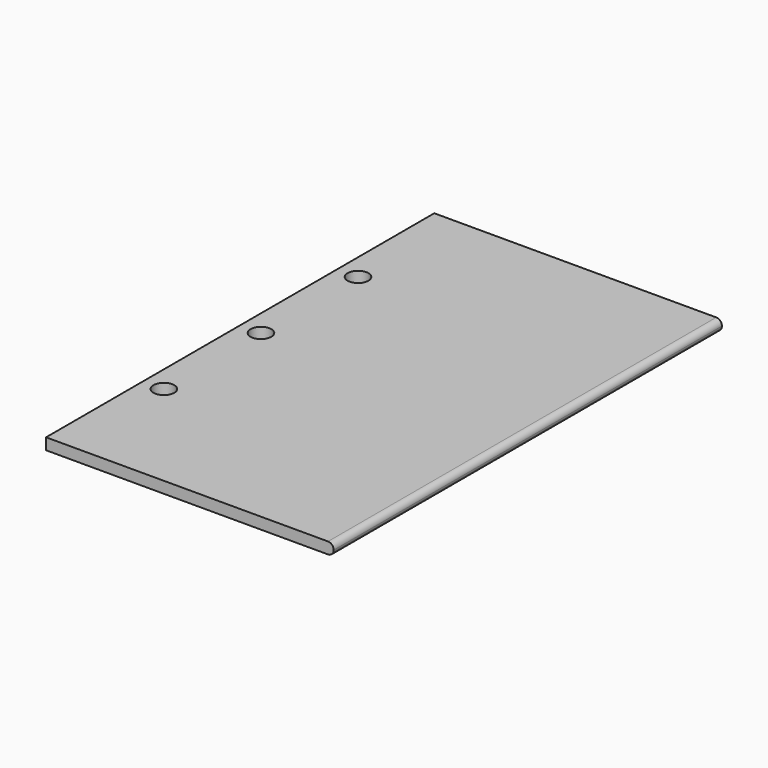
from build123d import *

# Parameters (mm, degrees)
F0_W     = 830
F0_H     = 1400
F1_DEPTH = 33
F2_R     = 16.49999
F4_D     = 60


# Not quite as in the source:
# - a fillet or chamfer is up to 0.001 mm smaller than in the source, because OpenCascade refuses the exact size


with BuildPart() as f1:
    # F0 (on Top) → F1 (new body)
    with BuildSketch(Plane.XY):
        with Locations((354.4717663527, -700)):
            Rectangle(F0_W, F0_H)
    extrude(amount=F1_DEPTH)

    # F2 (radius 16.5 in the source; OpenCascade refuses exactly that, so slightly less here)
    f2_edges = [f1.edges().sort_by_distance(p)[0] for p in [
        (769.471766, -700, 33),
        (769.471766, -700, 0),
    ]]
    fillet(f2_edges, radius=F2_R)

    # F4 (through all)
    with Locations(Plane.XY.offset(33)):
        with Locations((-0.5282336473, -1050), (-0.5282336473, -700), (-0.5282336473, -350)):
            Hole(F4_D / 2)


solid = f1.part
